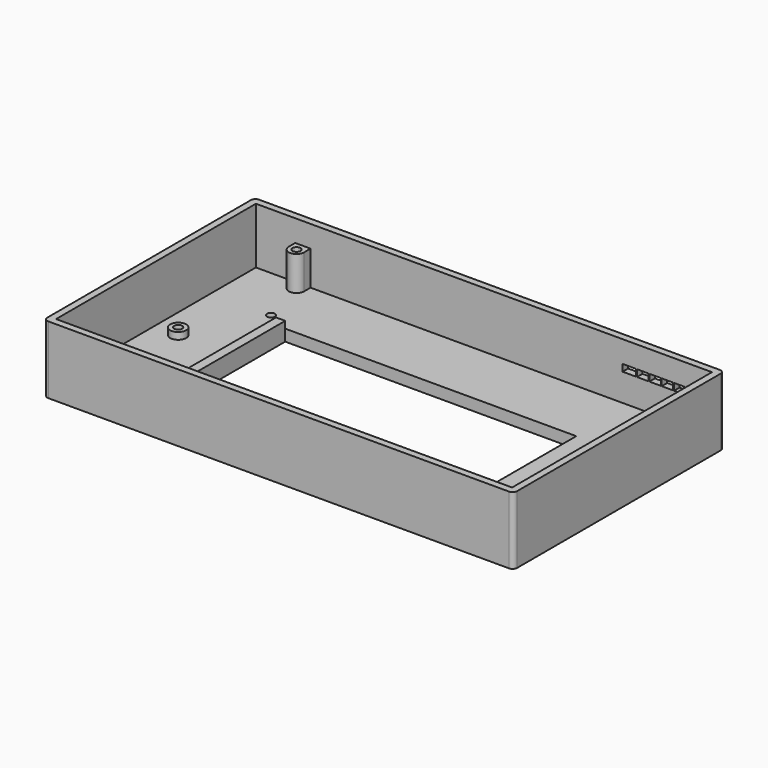
from build123d import *

# Parameters (mm, degrees)
F0_W      = 205
F0_H      = 115
F1_DEPTH  = 5
F2_R      = 1.75
F3_DEPTH  = 25
F4_W      = 127
F4_H      = 57
F5_DEPTH  = 25
F7_DEPTH  = 15
F9_DEPTH  = 3
F10_W     = 4
F10_H     = 57
F11_DEPTH = 3
F12_R     = 1.75
F13_DEPTH = 25
F14_R     = 1.75
F15_DEPTH = 25
F16_R     = 1.75
F17_DEPTH = 25
F18_R     = 1.75
F19_DEPTH = 25
F20_R     = 1.75
F21_DEPTH = 5
F22_W     = 168.3
F22_H     = 3
F23_DEPTH = 24.5
F24_R     = 2
F25_W     = 27
F25_H     = 3
F26_DEPTH = 25
F27_W     = 0.4
F27_H     = 3
F28_DEPTH = 3
F29_W     = 6.7
F29_H     = 3
F30_DEPTH = 9.5
F31_W     = 6.7
F31_H     = 3
F32_DEPTH = 9.5
F33_W     = 6.7
F33_H     = 3
F34_DEPTH = 9.5
F35_W     = 6.7
F35_H     = 3
F36_DEPTH = 9.5


# Not quite as in the source:
# - a feature names something its author has since deleted; it is built from what else it names


with BuildPart() as f1:
    # F0 (on Top) → F1 (new body)
    with BuildSketch(Plane.XY):
        with Locations((0.1253969967, -22.0995221115)):
            Rectangle(F0_W, F0_H)
    extrude(amount=F1_DEPTH)

    # F2 (on face) → F3 (cut)
    with BuildSketch(Plane(origin=(0, 0, 0), x_dir=(1, 0, 0), z_dir=(0, 0, -1))):
        with Locations((-73.3746030033, 59.5995221115)):
            Circle(F2_R)
        with Locations((-73.3746030033, -8.1444778885)):
            Circle(F2_R)
        with Locations((73.6253969967, 59.5995221115)):
            Circle(F2_R)
        with Locations((73.6253969967, -8.1444778885)):
            Circle(F2_R)
    extrude(amount=-F3_DEPTH, mode=Mode.SUBTRACT)

    # F4 (on face) → F5 (cut)
    with BuildSketch(Plane(origin=(0, 0, 0), x_dir=(1, 0, 0), z_dir=(0, 0, -1))):
        with Locations((0.1253969967, 25.0995221115)):
            Rectangle(F4_W, F4_H)
    extrude(amount=-F5_DEPTH, mode=Mode.SUBTRACT)

    # F6 (on face) → F7 (join)
    with BuildSketch(Plane.XY.offset(5)):
        with BuildLine():
            Line((96.1253969967, -73.0995221115), (99.4753969967, -73.0995221115))
            ThreePointArc((99.4753969967, -73.0995221115), (96.1253969967, -69.7495221115), (92.7753969967, -73.0995221115))
            Line((92.7753969967, -73.0995221115), (96.1253969967, -73.0995221115))
        make_face()
        with BuildLine():
            ThreePointArc((92.7753969967, -73.0995221115), (96.1253969967, -76.4495221115), (99.4753969967, -73.0995221115))
            Line((99.4753969967, -73.0995221115), (96.1253969967, -73.0995221115))
            Line((96.1253969967, -73.0995221115), (92.7753969967, -73.0995221115))
        make_face()
        with BuildLine():
            Line((-78.8746030033, -73.0995221115), (-75.5246030033, -73.0995221115))
            ThreePointArc((-75.5246030033, -73.0995221115), (-78.8746030033, -69.7495221115), (-82.2246030033, -73.0995221115))
            Line((-82.2246030033, -73.0995221115), (-78.8746030033, -73.0995221115))
        make_face()
        with BuildLine():
            ThreePointArc((-82.2246030033, -73.0995221115), (-78.8746030033, -76.4495221115), (-75.5246030033, -73.0995221115))
            Line((-75.5246030033, -73.0995221115), (-78.8746030033, -73.0995221115))
            Line((-78.8746030033, -73.0995221115), (-82.2246030033, -73.0995221115))
        make_face()
        with BuildLine():
            Line((96.1253969967, 28.9004778885), (99.4753969967, 28.9004778885))
            ThreePointArc((99.4753969967, 28.9004778885), (96.1253969967, 32.2504778885), (92.7753969967, 28.9004778885))
            Line((92.7753969967, 28.9004778885), (96.1253969967, 28.9004778885))
        make_face()
        with BuildLine():
            ThreePointArc((92.7753969967, 28.9004778885), (96.1253969967, 25.5504778885), (99.4753969967, 28.9004778885))
            Line((99.4753969967, 28.9004778885), (96.1253969967, 28.9004778885))
            Line((96.1253969967, 28.9004778885), (92.7753969967, 28.9004778885))
        make_face()
        with BuildLine():
            ThreePointArc((-82.2246030033, 28.9004778885), (-78.8746030033, 25.5504778885), (-75.5246030033, 28.9004778885))
            ThreePointArc((-75.5246030033, 28.9004778885), (-78.8746030033, 32.2504778885), (-82.2246030033, 28.9004778885))
        make_face()
        with BuildLine():
            Line((-82.2246030033, -79.5995221115), (-75.5246030033, -79.5995221115))
            Line((-75.5246030033, -79.5995221115), (-75.5246030033, -73.0995221115))
            ThreePointArc((-75.5246030033, -73.0995221115), (-78.8746030033, -76.4495221115), (-82.2246030033, -73.0995221115))
            Line((-82.2246030033, -73.0995221115), (-82.2246030033, -79.5995221115))
        make_face()
        with BuildLine():
            Line((-75.5246030033, 28.9004778885), (-75.5246030033, 35.4004778885))
            Line((-75.5246030033, 35.4004778885), (-82.2246030033, 35.4004778885))
            Line((-82.2246030033, 35.4004778885), (-82.2246030033, 28.9004778885))
            ThreePointArc((-82.2246030033, 28.9004778885), (-78.8746030033, 32.2504778885), (-75.5246030033, 28.9004778885))
        make_face()
        with BuildLine():
            Line((99.4753969967, 28.9004778885), (99.4753969967, 35.4004778885))
            Line((99.4753969967, 35.4004778885), (92.7753969967, 35.4004778885))
            Line((92.7753969967, 35.4004778885), (92.7753969967, 28.9004778885))
            ThreePointArc((92.7753969967, 28.9004778885), (96.1253969967, 32.2504778885), (99.4753969967, 28.9004778885))
        make_face()
        with BuildLine():
            Line((99.4753969967, -79.5995221115), (99.4753969967, -73.0995221115))
            ThreePointArc((99.4753969967, -73.0995221115), (96.1253969967, -76.4495221115), (92.7753969967, -73.0995221115))
            Line((92.7753969967, -73.0995221115), (92.7753969967, -79.5995221115))
            Line((92.7753969967, -79.5995221115), (99.4753969967, -79.5995221115))
        make_face()
    extrude(amount=F7_DEPTH)

    # F8 (on face) → F9 (join)
    with BuildSketch(Plane.XY.offset(5)):
        with BuildLine():
            ThreePointArc((-92.3746030033, -23.0995221115), (-88.8746030033, -26.5995221115), (-85.3746030033, -23.0995221115))
            Line((-85.3746030033, -23.0995221115), (-92.3746030033, -23.0995221115))
        make_face()
        with BuildLine():
            Line((-92.3746030033, -23.0995221115), (-85.3746030033, -23.0995221115))
            ThreePointArc((-85.3746030033, -23.0995221115), (-88.8746030033, -19.5995221115), (-92.3746030033, -23.0995221115))
        make_face()
    extrude(amount=F9_DEPTH)

    # F10 (on face) → F11 (join)
    with BuildSketch(Plane.XY.offset(5)):
        with Locations((-65.3746030033, -25.0995221115)):
            Rectangle(F10_W, F10_H)
    extrude(amount=F11_DEPTH)

    # F12 (on face) → F13 (cut)
    with BuildSketch(Plane.XY.offset(20)):
        with Locations((-78.8746030033, -73.0995221115)):
            Circle(F12_R)
    extrude(amount=-F13_DEPTH, mode=Mode.SUBTRACT)

    # F14 (on face) → F15 (cut)
    with BuildSketch(Plane.XY.offset(20)):
        with Locations((-78.8746030033, 28.9004778885)):
            Circle(F14_R)
    extrude(amount=-F15_DEPTH, mode=Mode.SUBTRACT)

    # F16 (on face) → F17 (cut)
    with BuildSketch(Plane.XY.offset(20)):
        with Locations((96.1253969967, -73.0995221115)):
            Circle(F16_R)
    extrude(amount=-F17_DEPTH, mode=Mode.SUBTRACT)

    # F18 (on face) → F19 (cut)
    with BuildSketch(Plane.XY.offset(20)):
        with Locations((96.1253969967, 28.9004778885)):
            Circle(F18_R)
    extrude(amount=-F19_DEPTH, mode=Mode.SUBTRACT)

    # F20 (on face) → F21 (cut)
    with BuildSketch(Plane.XY.offset(8)):
        with Locations((-88.8746030033, -23.0995221115)):
            Circle(F20_R)
    extrude(amount=-F21_DEPTH, mode=Mode.SUBTRACT)

    # F22 (on face) → F23 (join)
    with BuildSketch(Plane.XY.offset(5)):
        Polygon((99.4753969967, -79.5995221115), (102.6253969967, -79.5995221115), (102.6253969967, 35.4004778885), (99.4753969967, 35.4004778885), (99.4753969967, 32.4004778885), (99.6253969967, 32.4004778885), (99.6253969967, -76.5995221115), (99.4753969967, -76.5995221115), align=None)
        Polygon((-102.3746030033, -79.5995221115), (-82.2246030033, -79.5995221115), (-82.2246030033, -76.5995221115), (-99.3746030033, -76.5995221115), (-99.3746030033, 32.4004778885), (-82.2246030033, 32.4004778885), (-82.2246030033, 35.4004778885), (-102.3746030033, 35.4004778885), align=None)
        with Locations((8.6253969967, -78.0995221115)):
            Rectangle(F22_W, F22_H)
        with Locations((8.6253969967, 33.9004778885)):
            Rectangle(F22_W, F22_H)
    extrude(amount=F23_DEPTH)

    # F24
    f24_edges = [f1.edges().sort_by_distance(p)[0] for p in [
        (-102.374603, -79.599522, 14.75),
        (102.625397, -79.599522, 14.75),
        (102.625397, 35.400478, 14.75),
        (-102.374603, 35.400478, 14.75),
    ]]
    fillet(f24_edges, radius=F24_R)

    # F25 (on face) → F26 (cut)
    with BuildSketch(Plane.XZ.offset(-32.4004778885)):
        with Locations((74.1253969967, 18.5)):
            Rectangle(F25_W, F25_H)
    extrude(amount=-F26_DEPTH, mode=Mode.SUBTRACT)

    # F27 (on face) → F28 (join)
    with BuildSketch(Plane.XY.offset(17)):
        with Locations((82.9253969967, 33.9004778885)):
            Rectangle(F27_W, F27_H)
        with Locations((77.5253969967, 33.9004778885)):
            Rectangle(F27_W, F27_H)
        with Locations((72.1253969967, 33.9004778885)):
            Rectangle(F27_W, F27_H)
        with Locations((66.7253969967, 33.9004778885)):
            Rectangle(F27_W, F27_H)
    extrude(amount=F28_DEPTH)

    # F29 (on face) → F30 (join)
    with BuildSketch(Plane.XY.offset(20)):
        with Locations((-78.8746030033, -78.0995221115)):
            Rectangle(F29_W, F29_H)
    extrude(amount=F30_DEPTH)

    # F31 (on face) → F32 (join)
    with BuildSketch(Plane.XY.offset(20)):
        with Locations((96.1253969967, -78.0995221115)):
            Rectangle(F31_W, F31_H)
    extrude(amount=F32_DEPTH)

    # F33 (on face) → F34 (join)
    with BuildSketch(Plane.XY.offset(20)):
        with Locations((96.1253969967, 33.9004778885)):
            Rectangle(F33_W, F33_H)
    extrude(amount=F34_DEPTH)

    # F35 (on face) → F36 (join)
    with BuildSketch(Plane.XY.offset(20)):
        with Locations((-78.8746030033, 33.9004778885)):
            Rectangle(F35_W, F35_H)
    extrude(amount=F36_DEPTH)


solid = f1.part
